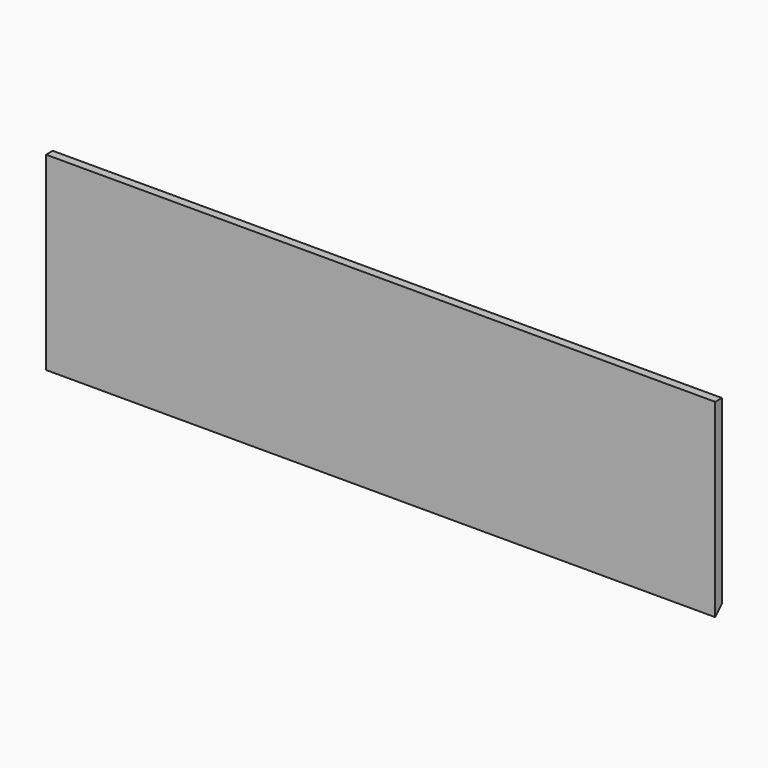
from build123d import *

# Parameters (mm, degrees)
F0_W     = 1524
F0_H     = 431.8
F1_DEPTH = 19.05
F2_SIZE  = 19.04999


# Not quite as in the source:
# - a fillet or chamfer is up to 0.001 mm smaller than in the source, because OpenCascade refuses the exact size


with BuildPart() as f1:
    # F0 (on Front) → F1 (new body)
    with BuildSketch(Plane.XZ):
        with Locations((762, 215.9)):
            Rectangle(F0_W, F0_H)
    extrude(amount=F1_DEPTH)

    # F2 (size 19.05 in the source; OpenCascade refuses exactly that, so slightly less here)
    f2_edges = [f1.edges().sort_by_distance(p)[0] for p in [
        (762, 0, 0),
    ]]
    chamfer(f2_edges, length=F2_SIZE)


solid = f1.part
